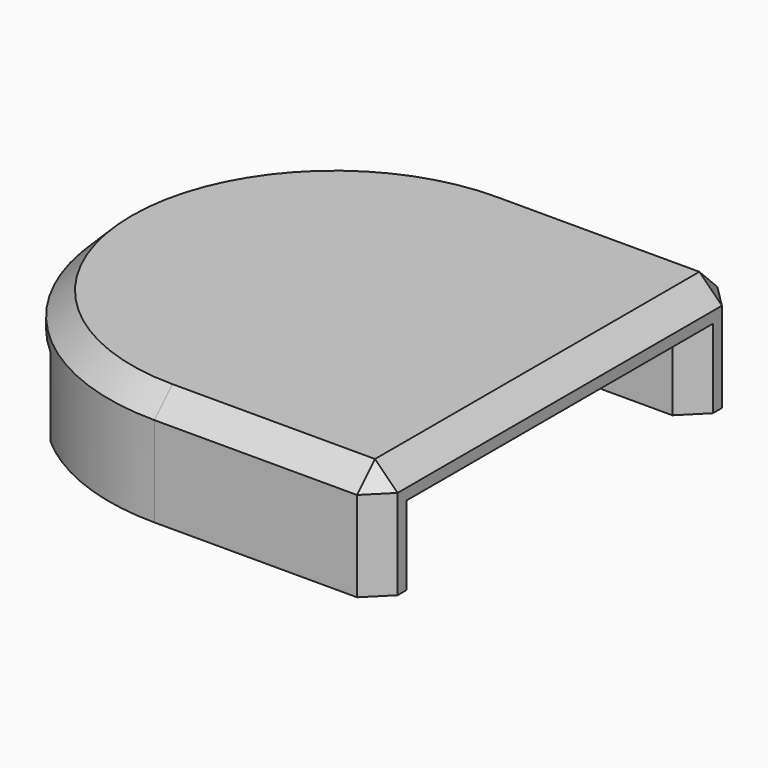
from build123d import *

# Parameters (mm, degrees)
F0_W     = 40
F0_H     = 40
F1_DEPTH = 3
F2_W     = 40
F2_H     = 5
F3_DEPTH = 7
F4_R     = 19.99999
F5_SIZE  = 2


# Not quite as in the source:
# - a fillet or chamfer is up to 0.001 mm smaller than in the source, because OpenCascade refuses the exact size


with BuildPart() as f1:
    # F0 (on Top) → F1 (new body)
    with BuildSketch(Plane.XY):
        Rectangle(F0_W, F0_H)
    extrude(amount=F1_DEPTH)

    # F2 (on face) → F3 (join)
    with BuildSketch(Plane(origin=(0, 0, 0), x_dir=(1, 0, 0), z_dir=(0, 0, -1))):
        with Locations((0, 17.5)):
            Rectangle(F2_W, F2_H)
        with Locations((0, -17.5)):
            Rectangle(F2_W, F2_H)
    extrude(amount=F3_DEPTH)

    # F4 (radius 20 in the source; OpenCascade refuses exactly that, so slightly less here)
    f4_edges = [f1.edges().sort_by_distance(p)[0] for p in [
        (-20, 20, -2),
        (-20, -20, -2),
    ]]
    fillet(f4_edges, radius=F4_R)

    # F5
    f5_edges = [f1.edges().sort_by_distance(p)[0] for p in [
        (-14.142139, -14.142139, 3),
        (20, -20, -2),
        (20, 0, 3),
        (20, 20, -2),
        (20, 15, -3.5),
        (20, -15, -3.5),
    ]]
    chamfer(f5_edges, length=F5_SIZE)


solid = f1.part
